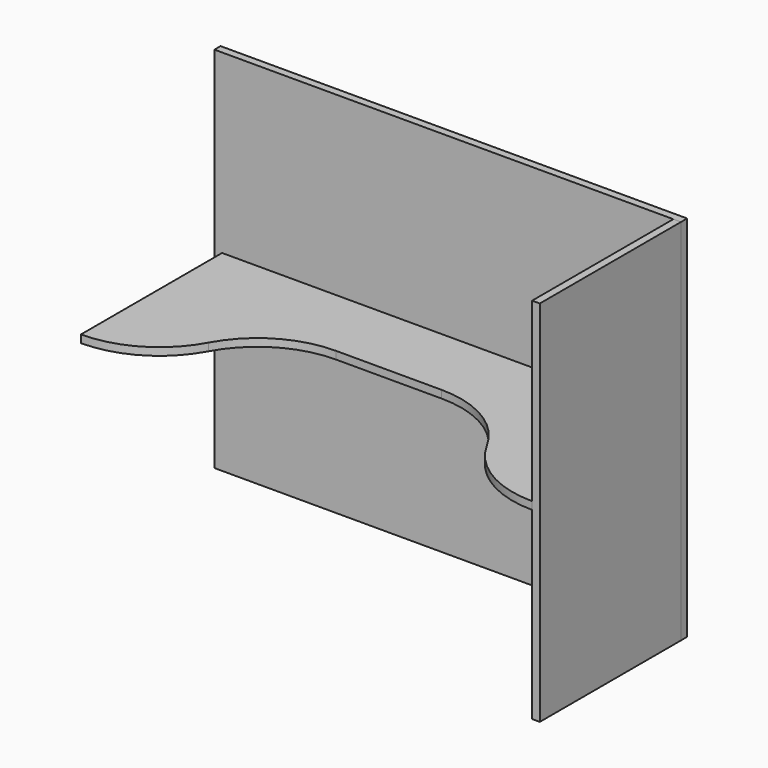
from build123d import *

# Parameters (mm, degrees)
F0_W     = 965.2
F0_H     = 762
F1_DEPTH = 15.875
F2_W     = 365.125
F2_H     = 762
F3_DEPTH = 15.875
F5_DEPTH = 15.875


with BuildPart() as f1:
    # F0 (on Front) → F1 (new body)
    with BuildSketch(Plane.XZ):
        Rectangle(F0_W, F0_H)
    extrude(amount=-F1_DEPTH)


with BuildPart() as f3:
    # F2 (on face) → F3 (new body)
    with BuildSketch(Plane.YZ.offset(482.6)):
        with Locations((-182.5625, 0)):
            Rectangle(F2_W, F2_H)
    extrude(amount=-F3_DEPTH)


with BuildPart() as f5:
    # F4 (on Top) → F5 (new body)
    with BuildSketch(Plane.XY):
        with BuildLine():
            Line((466.725, -365.125), (466.725, 0))
            Line((466.725, 0), (0, 0))
            Line((0, 0), (0, -152.4))
            Line((0, -152.4), (109.4422626966, -152.4))
            ThreePointArc((109.4422626966, -152.4), (213.3962428994, -181.0038660222), (288.0836313483, -258.7625))
            ThreePointArc((288.0836313483, -258.7625), (362.7710197972, -336.5211339778), (466.725, -365.125))
        make_face()
    extrude(amount=F5_DEPTH)

    # F6: F5 across plane


with BuildPart() as f5_1:
    add(f5.part)
    add(f5.part.mirror(Plane.YZ))


solid = Compound([f1.part, f3.part, f5_1.part])
